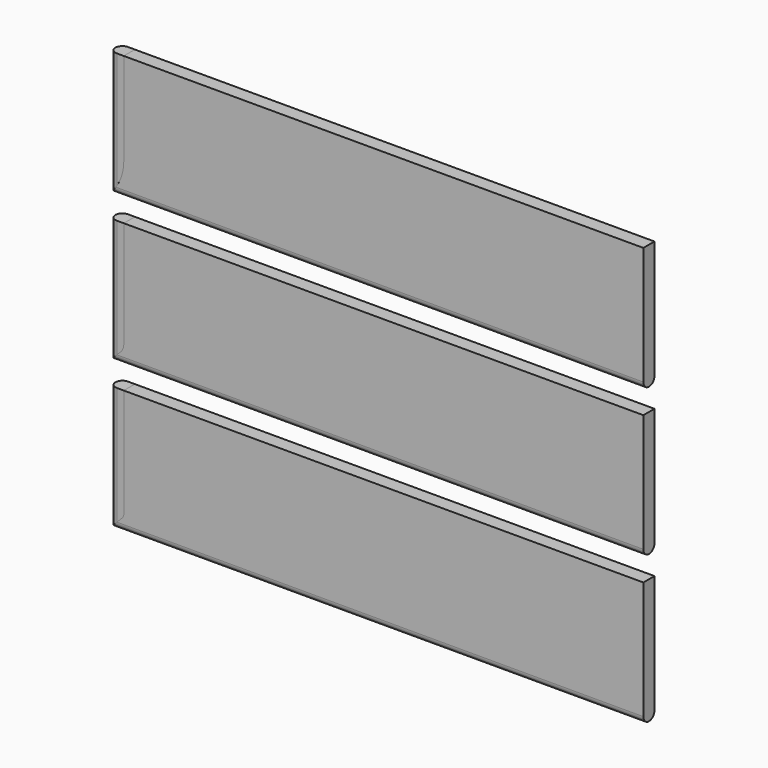
from build123d import *

# Parameters (mm, degrees)
F1_DEPTH = 31.75
F2_DEPTH = 31.75
F3_R     = 15.87499
F3_2_R   = 15.87499
F3_3_R   = 15.87499
F3_4_R   = 15.87499
F3_5_R   = 15.87499
F3_6_R   = 15.87499


# Not quite as in the source:
# - a fillet or chamfer is up to 0.001 mm smaller than in the source, because OpenCascade refuses the exact size


with BuildPart() as f1:
    # F0 (on Front) → F1 (new body)
    with BuildSketch(Plane.XZ):
        with BuildLine():
            Line((623.6085797757, 69.8951120117), (-563.8414202243, 69.8951120117))
            Line((-563.8414202243, 69.8951120117), (-563.8414202243, -142.074555243))
            ThreePointArc((-563.8414202243, -142.074555243), (-572.1158610243, -182.2354815272), (-595.5914202243, -215.8548879883))
            Line((-595.5914202243, -215.8548879883), (623.6085797757, -215.8548879883))
            Line((623.6085797757, -215.8548879883), (623.6085797757, 69.8951120117))
        make_face()
    extrude(amount=F1_DEPTH)

    # F3#6 (radius 15.875 in the source; OpenCascade refuses exactly that, so slightly less here)
    f3_6_edges = [f1.edges().sort_by_distance(p)[0] for p in [
        (14.00858, -31.75, -215.854888),
        (14.00858, 0, -215.854888),
    ]]
    fillet(f3_6_edges, radius=F3_6_R)


with BuildPart() as f1b:
    # F0 (on Front) → F1, piece 2 (new body)
    with BuildSketch(Plane.XZ):
        with BuildLine():
            Line((623.6085797757, -266.6548879883), (-563.8414202243, -266.6548879883))
            Line((-563.8414202243, -266.6548879883), (-563.8414202243, -510.133863504))
            ThreePointArc((-563.8414202243, -510.133863504), (-565.7748800985, -519.8540226861), (-571.2809079822, -528.0943757462))
            Line((-571.2809079822, -528.0943757462), (-595.5914202243, -552.4048879883))
            Line((-595.5914202243, -552.4048879883), (623.6085797757, -552.4048879883))
            Line((623.6085797757, -552.4048879883), (623.6085797757, -266.6548879883))
        make_face()
    extrude(amount=F1_DEPTH)

    # F3#3 (radius 15.875 in the source; OpenCascade refuses exactly that, so slightly less here)
    f3_3_edges = [f1b.edges().sort_by_distance(p)[0] for p in [
        (14.00858, -31.75, -552.404888),
        (14.00858, 0, -552.404888),
    ]]
    fillet(f3_3_edges, radius=F3_3_R)


with BuildPart() as f1c:
    # F0 (on Front) → F1, piece 3 (new body)
    with BuildSketch(Plane.XZ):
        with BuildLine():
            Line((623.6085797757, -603.2048879883), (-563.8414202243, -603.2048879883))
            Line((-563.8414202243, -603.2048879883), (-563.8414202243, -851.9443757462))
            ThreePointArc((-563.8414202243, -851.9443757462), (-564.8081501614, -856.8044553372), (-567.5611641032, -860.9246318672))
            Line((-567.5611641032, -860.9246318672), (-595.5914202243, -888.9548879883))
            Line((-595.5914202243, -888.9548879883), (623.6085797757, -888.9548879883))
            Line((623.6085797757, -888.9548879883), (623.6085797757, -603.2048879883))
        make_face()
    extrude(amount=F1_DEPTH)

    # F3 (radius 15.875 in the source; OpenCascade refuses exactly that, so slightly less here)
    f3_edges = [f1c.edges().sort_by_distance(p)[0] for p in [
        (14.00858, -31.75, -888.954888),
        (14.00858, 0, -888.954888),
    ]]
    fillet(f3_edges, radius=F3_R)


with BuildPart() as f2:
    # F0 (on Front) → F2 (new body)
    with BuildSketch(Plane.XZ):
        with BuildLine():
            Line((-563.8414202243, 69.8951120117), (-595.5914202243, 69.8951120117))
            Line((-595.5914202243, 69.8951120117), (-595.5914202243, -215.8548879883))
            ThreePointArc((-595.5914202243, -215.8548879883), (-572.1158610243, -182.2354815272), (-563.8414202243, -142.074555243))
            Line((-563.8414202243, -142.074555243), (-563.8414202243, 69.8951120117))
        make_face()
    extrude(amount=F2_DEPTH)

    # F3#5 (radius 15.875 in the source; OpenCascade refuses exactly that, so slightly less here)
    f3_5_edges = [f2.edges().sort_by_distance(p)[0] for p in [
        (-595.59142, -31.75, -72.979888),
        (-595.59142, 0, -72.979888),
    ]]
    fillet(f3_5_edges, radius=F3_5_R)


with BuildPart() as f2b:
    # F0 (on Front) → F2, piece 2 (new body)
    with BuildSketch(Plane.XZ):
        with BuildLine():
            Line((-563.8414202243, -266.6548879883), (-595.5914202243, -266.6548879883))
            Line((-595.5914202243, -266.6548879883), (-595.5914202243, -552.4048879883))
            Line((-595.5914202243, -552.4048879883), (-571.2809079822, -528.0943757462))
            ThreePointArc((-571.2809079822, -528.0943757462), (-565.7748800985, -519.8540226861), (-563.8414202243, -510.133863504))
            Line((-563.8414202243, -510.133863504), (-563.8414202243, -266.6548879883))
        make_face()
    extrude(amount=F2_DEPTH)

    # F3#4 (radius 15.875 in the source; OpenCascade refuses exactly that, so slightly less here)
    f3_4_edges = [f2b.edges().sort_by_distance(p)[0] for p in [
        (-595.59142, -31.75, -409.529888),
        (-595.59142, 0, -409.529888),
    ]]
    fillet(f3_4_edges, radius=F3_4_R)


with BuildPart() as f2c:
    # F0 (on Front) → F2, piece 3 (new body)
    with BuildSketch(Plane.XZ):
        with BuildLine():
            Line((-563.8414202243, -603.2048879883), (-595.5914202243, -603.2048879883))
            Line((-595.5914202243, -603.2048879883), (-595.5914202243, -888.9548879883))
            Line((-595.5914202243, -888.9548879883), (-567.5611641032, -860.9246318672))
            ThreePointArc((-567.5611641032, -860.9246318672), (-564.8081501614, -856.8044553372), (-563.8414202243, -851.9443757462))
            Line((-563.8414202243, -851.9443757462), (-563.8414202243, -603.2048879883))
        make_face()
    extrude(amount=F2_DEPTH)

    # F3#2 (radius 15.875 in the source; OpenCascade refuses exactly that, so slightly less here)
    f3_2_edges = [f2c.edges().sort_by_distance(p)[0] for p in [
        (-595.59142, -31.75, -746.079888),
        (-595.59142, 0, -746.079888),
    ]]
    fillet(f3_2_edges, radius=F3_2_R)


solid = Compound([f1.part, f1b.part, f1c.part, f2.part, f2b.part, f2c.part])
